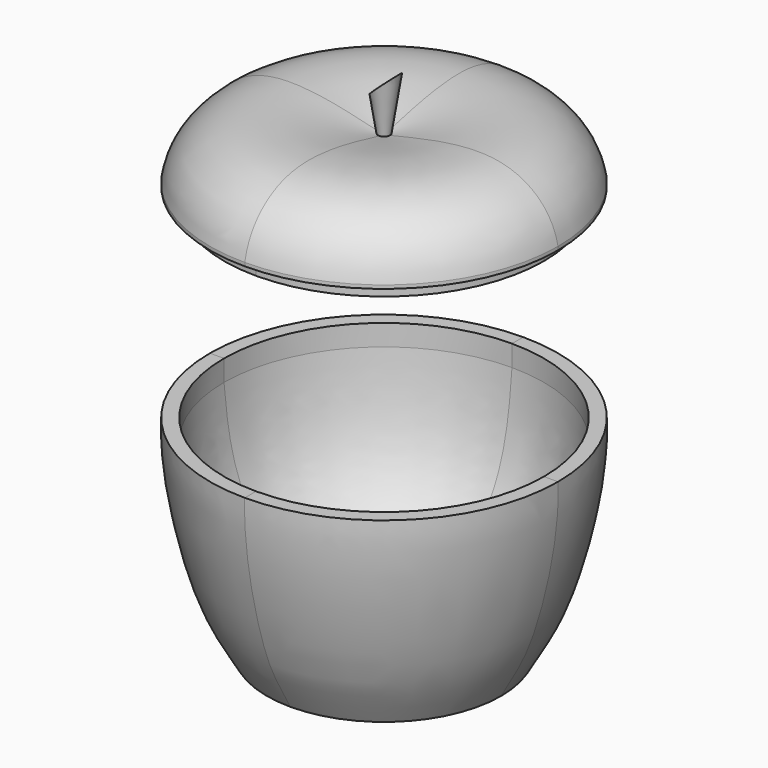
from build123d import *

# Parameters (mm, degrees)
F1_W     = 50
F1_H     = 50
F2_DEPTH = 125
F3_DEPTH = 125
F6_DEPTH = 12.5


# Not quite as in the source:
# - a feature names something its author has since deleted; it is built from what else it names


with BuildPart() as f2:
    # F1 (on Top) → F2 (new body, symmetric)
    with BuildSketch(Plane.XY):
        with Locations((-25, 25)):
            Rectangle(F1_W, F1_H)
    extrude(amount=F2_DEPTH, both=True)


with BuildPart() as f2b:
    # F1 (on Top) → F2, piece 2 (new body, symmetric)
    with BuildSketch(Plane.XY):
        with Locations((25, -25)):
            Rectangle(F1_W, F1_H)
    extrude(amount=F2_DEPTH, both=True)


with BuildPart() as f3:
    # F1 (on Top) → F3 (new body, symmetric)
    with BuildSketch(Plane.XY):
        with Locations((25, 25)):
            Rectangle(F1_W, F1_H)
    extrude(amount=F3_DEPTH, both=True)


with BuildPart() as f3b:
    # F1 (on Top) → F3, piece 2 (new body, symmetric)
    with BuildSketch(Plane.XY):
        with Locations((-25, -25)):
            Rectangle(F1_W, F1_H)
    extrude(amount=F3_DEPTH, both=True)


with BuildPart() as f4_tool:
    # F0 (on Front) → F4 (revolve)
    with BuildSketch(Plane.XZ):
        with BuildLine():
            Line((49.438945465, 86.7833935618), (49.438945465, 87.7833935618))
            add(Edge.make_bspline(
                [(49.438945465, 87.7833935618), (47.8022624163, 96.2052666264), (33.9687495317, 108.4631394379), (10.3452695599, 101.9952321233), (1.6933184816, 99.9940857291)],
                knots=[0, 0, 0, 0, 0.4591296552, 1, 1, 1, 1], degree=3))
            Line((1.6933184816, 99.9940857291), (0, 99.9940857291))
            Line((0, 99.9940857291), (0, 97.6326140165))
            add(Edge.make_bspline(
                [(42.438945465, 87.7833935618), (42.0025324422, 90.6852536777), (38.8255918779, 98.4192460488), (19.6814191356, 98.3476648556), (7.3225652051, 97.5483304261), (0, 97.6326140165)],
                knots=[0, 0, 0, 0, 0.2597363864, 0.6121745345, 1, 1, 1, 1], degree=3))
            Line((42.438945465, 87.7833935618), (42.438945465, 82.7833935618))
            Line((42.438945465, 82.7833935618), (45.438945465, 82.7833935618))
            Line((45.438945465, 82.7833935618), (45.438945465, 86.7833935618))
            Line((45.438945465, 86.7833935618), (49.438945465, 86.7833935618))
        make_face()
        with BuildLine():
            Line((0, -20.4283881187), (0, -24.9324262887))
            Line((0, -24.9324262887), (26, -24.9324262887))
            Line((26, -24.9324262887), (24.6602540378, -29.9324262887))
            Line((24.6602540378, -29.9324262887), (33.26735273, -29.9324262887))
            add(Edge.make_bspline(
                [(33.26735273, -29.9324262887), (38.2139571011, -21.5028394014), (43.0940634091, -13.2385249434), (50, 15.6583895273), (49.438945465, 28.8983398523)],
                knots=[0, 0, 0, 0, 0.4202473193, 1, 1, 1, 1], degree=3))
            Line((49.438945465, 28.8983398523), (45.438945465, 28.8983398523))
            Line((45.438945465, 28.8983398523), (45.438945465, 22.8983398523))
            add(Edge.make_bspline(
                [(45.438945465, 22.8983398523), (44.1422413956, 6.9057072158), (39.7512452022, -6.6381642264), (25.0377642283, -21.7866553606), (12.9342993017, -20.1565072632), (0, -20.4283881187)],
                knots=[0, 0, 0, 0, 0.3834354123, 0.6554833814, 1, 1, 1, 1], degree=3))
        make_face()
    revolve(axis=Axis((0, 0, 78.9686217904), (0, 0, 1)))


with BuildPart() as f2_1:
    add(f2.part)

    # F4: intersect by f4_tool
    add(f4_tool.part, mode=Mode.INTERSECT)


with BuildPart() as f2b_1:
    add(f2b.part)

    # F4: intersect by f4_tool
    add(f4_tool.part, mode=Mode.INTERSECT)


with BuildPart() as f3_1:
    add(f3.part)

    # F4: intersect by f4_tool
    add(f4_tool.part, mode=Mode.INTERSECT)


with BuildPart() as f3b_1:
    add(f3b.part)

    # F4: intersect by f4_tool
    add(f4_tool.part, mode=Mode.INTERSECT)


with BuildPart() as f5:
    # F0 (on Front) → F5 (revolve)
    with BuildSketch(Plane.XZ):
        Polygon((0, 99.9940857291), (1.6933184816, 99.9940857291), (4.15784137, 115.925386548), (0, 112.0865344652), align=None)
        Polygon((0, 112.0865344652), (4.15784137, 115.925386548), (0, 115.925386548), align=None)
    revolve(axis=Axis((0, 0, 78.9686217904), (0, 0, 1)))

    # F0 (on Front) → F6 (cut, symmetric)
    with BuildSketch(Plane.XZ):
        Polygon((0, 112.0865344652), (4.15784137, 115.925386548), (0, 115.925386548), align=None)
        Polygon((0, 112.0865344652), (0, 115.925386548), (-7.2805839591, 115.925386548), (-7.2805839591, 105.3645163774), align=None)
    extrude(amount=F6_DEPTH, both=True, mode=Mode.SUBTRACT)


solid = Compound([f2_1.part, f2b_1.part, f3_1.part, f3b_1.part, f5.part])
